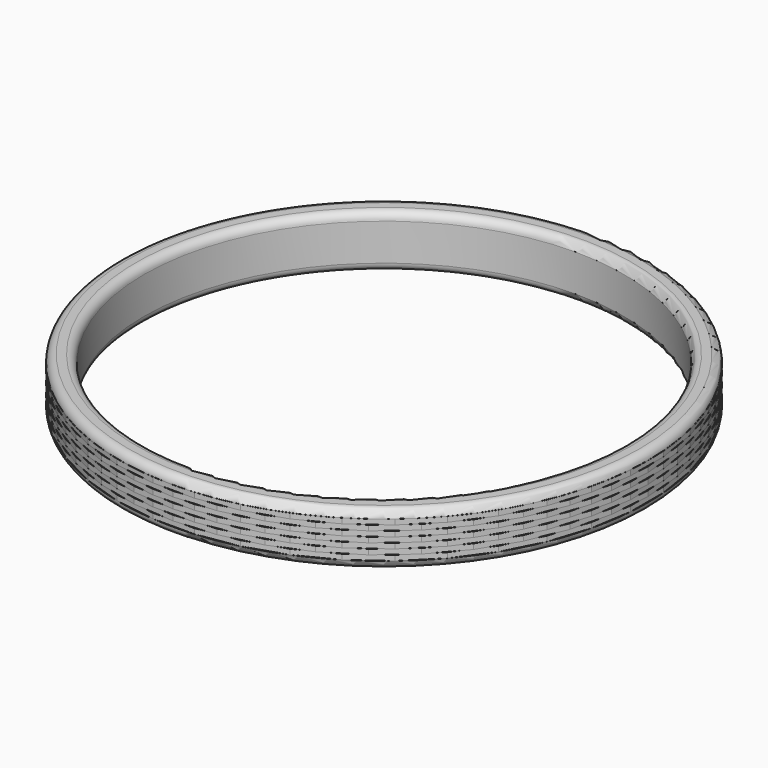
from build123d import *

# Parameters (mm, degrees)
F2_DEPTH  = 0.1
F4_DEPTH  = 0.2
F6_DEPTH  = 0.2
F8_DEPTH  = 0.2
F9_R      = 10
F10_DEPTH = 0.3
F0_R      = 9.095
F12_DEPTH = 5
F13_R     = 0.29999


# Not quite as in the source:
# - a fillet or chamfer is up to 0.001 mm smaller than in the source, because OpenCascade refuses the exact size


with BuildPart() as f2:
    # F1 (on Top) → F2 (new body, symmetric)
    with BuildSketch(Plane.XY):
        Polygon((9.876883406, -1.5643446504), (10, 0), (9.876883406, 1.5643446504), (9.510565163, 3.0901699437), (8.9100652419, 4.5399049974), (8.0901699437, 5.8778525229), (7.0710678119, 7.0710678119), (5.8778525229, 8.0901699437), (4.5399049974, 8.9100652419), (3.0901699437, 9.510565163), (1.5643446504, 9.876883406), (0, 10), (-1.5643446504, 9.876883406), (-3.0901699437, 9.510565163), (-4.5399049974, 8.9100652419), (-5.8778525229, 8.0901699437), (-7.0710678119, 7.0710678119), (-8.0901699437, 5.8778525229), (-8.9100652419, 4.5399049974), (-9.510565163, 3.0901699437), (-9.876883406, 1.5643446504), (-10, 0), (-9.876883406, -1.5643446504), (-9.510565163, -3.0901699437), (-8.9100652419, -4.5399049974), (-8.0901699437, -5.8778525229), (-7.0710678119, -7.0710678119), (-5.8778525229, -8.0901699437), (-4.5399049974, -8.9100652419), (-3.0901699437, -9.510565163), (-1.5643446504, -9.876883406), (0, -10), (1.5643446504, -9.876883406), (3.0901699437, -9.510565163), (4.5399049974, -8.9100652419), (5.8778525229, -8.0901699437), (7.0710678119, -7.0710678119), (8.0901699437, -5.8778525229), (8.9100652419, -4.5399049974), (9.510565163, -3.0901699437), align=None)
    extrude(amount=F2_DEPTH, both=True)

    # F3 (on face) → F4 (join)
    with BuildSketch(Plane.XY.offset(0.1)):
        Polygon((9.723699204, 2.3344536386), (9.2387953251, 3.8268343237), (8.5264016435, 5.2249856472), (7.604059656, 6.4944804833), (6.4944804833, 7.604059656), (5.2249856472, 8.5264016435), (3.8268343237, 9.2387953251), (2.3344536386, 9.723699204), (0.7845909573, 9.9691733373), (-0.7845909573, 9.9691733373), (-2.3344536386, 9.723699204), (-3.8268343237, 9.2387953251), (-5.2249856472, 8.5264016435), (-6.4944804833, 7.604059656), (-7.604059656, 6.4944804833), (-8.5264016435, 5.2249856472), (-9.2387953251, 3.8268343237), (-9.723699204, 2.3344536386), (-9.9691733373, 0.7845909573), (-9.9691733373, -0.7845909573), (-9.723699204, -2.3344536386), (-9.2387953251, -3.8268343237), (-8.5264016435, -5.2249856472), (-7.604059656, -6.4944804833), (-6.4944804833, -7.604059656), (-5.2249856472, -8.5264016435), (-3.8268343237, -9.2387953251), (-2.3344536386, -9.723699204), (-0.7845909573, -9.9691733373), (0.7845909573, -9.9691733373), (2.3344536386, -9.723699204), (3.8268343237, -9.2387953251), (5.2249856472, -8.5264016435), (6.4944804833, -7.604059656), (7.604059656, -6.4944804833), (8.5264016435, -5.2249856472), (9.2387953251, -3.8268343237), (9.723699204, -2.3344536386), (9.9691733373, -0.7845909573), (9.9691733373, 0.7845909573), align=None)
    extrude(amount=F4_DEPTH)

    # F5 (on face) → F6 (join)
    with BuildSketch(Plane.XY.offset(0.3)):
        Polygon((9.876883406, -1.5643446504), (10, 0), (9.876883406, 1.5643446504), (9.510565163, 3.0901699437), (8.9100652419, 4.5399049974), (8.0901699437, 5.8778525229), (7.0710678119, 7.0710678119), (5.8778525229, 8.0901699437), (4.5399049974, 8.9100652419), (3.0901699437, 9.510565163), (1.5643446504, 9.876883406), (0, 10), (-1.5643446504, 9.876883406), (-3.0901699437, 9.510565163), (-4.5399049974, 8.9100652419), (-5.8778525229, 8.0901699437), (-7.0710678119, 7.0710678119), (-8.0901699437, 5.8778525229), (-8.9100652419, 4.5399049974), (-9.510565163, 3.0901699437), (-9.876883406, 1.5643446504), (-10, 0), (-9.876883406, -1.5643446504), (-9.510565163, -3.0901699437), (-8.9100652419, -4.5399049974), (-8.0901699437, -5.8778525229), (-7.0710678119, -7.0710678119), (-5.8778525229, -8.0901699437), (-4.5399049974, -8.9100652419), (-3.0901699437, -9.510565163), (-1.5643446504, -9.876883406), (0, -10), (1.5643446504, -9.876883406), (3.0901699437, -9.510565163), (4.5399049974, -8.9100652419), (5.8778525229, -8.0901699437), (7.0710678119, -7.0710678119), (8.0901699437, -5.8778525229), (8.9100652419, -4.5399049974), (9.510565163, -3.0901699437), align=None)
    extrude(amount=F6_DEPTH)

    # F7 (on face) → F8 (join)
    with BuildSketch(Plane.XY.offset(0.5)):
        Polygon((9.723699204, 2.3344536386), (9.2387953251, 3.8268343237), (8.5264016435, 5.2249856472), (7.604059656, 6.4944804833), (6.4944804833, 7.604059656), (5.2249856472, 8.5264016435), (3.8268343237, 9.2387953251), (2.3344536386, 9.723699204), (0.7845909573, 9.9691733373), (-0.7845909573, 9.9691733373), (-2.3344536386, 9.723699204), (-3.8268343237, 9.2387953251), (-5.2249856472, 8.5264016435), (-6.4944804833, 7.604059656), (-7.604059656, 6.4944804833), (-8.5264016435, 5.2249856472), (-9.2387953251, 3.8268343237), (-9.723699204, 2.3344536386), (-9.9691733373, 0.7845909573), (-9.9691733373, -0.7845909573), (-9.723699204, -2.3344536386), (-9.2387953251, -3.8268343237), (-8.5264016435, -5.2249856472), (-7.604059656, -6.4944804833), (-6.4944804833, -7.604059656), (-5.2249856472, -8.5264016435), (-3.8268343237, -9.2387953251), (-2.3344536386, -9.723699204), (-0.7845909573, -9.9691733373), (0.7845909573, -9.9691733373), (2.3344536386, -9.723699204), (3.8268343237, -9.2387953251), (5.2249856472, -8.5264016435), (6.4944804833, -7.604059656), (7.604059656, -6.4944804833), (8.5264016435, -5.2249856472), (9.2387953251, -3.8268343237), (9.723699204, -2.3344536386), (9.9691733373, -0.7845909573), (9.9691733373, 0.7845909573), align=None)
    extrude(amount=F8_DEPTH)

    # F9 (on face) → F10 (join)
    with BuildSketch(Plane.XY.offset(0.7)):
        Circle(F9_R)
    extrude(amount=F10_DEPTH)

    # F11: F2 across plane


with BuildPart() as f2_1:
    add(f2.part)
    add(f2.part.mirror(Plane.XY))

    # F0 (on Top) → F12 (cut, symmetric)
    with BuildSketch(Plane.XY):
        Circle(F0_R)
    extrude(amount=F12_DEPTH, both=True, mode=Mode.SUBTRACT)

    # F13 (radius 0.3 in the source; OpenCascade refuses exactly that, so slightly less here)
    f13_edges = [f2_1.edges().sort_by_distance(p)[0] for p in [
        (-10, 0, 1),
        (-9.095, 0, 1),
        (-10, 0, -1),
        (-9.095, 0, -1),
    ]]
    fillet(f13_edges, radius=F13_R)


solid = f2_1.part
